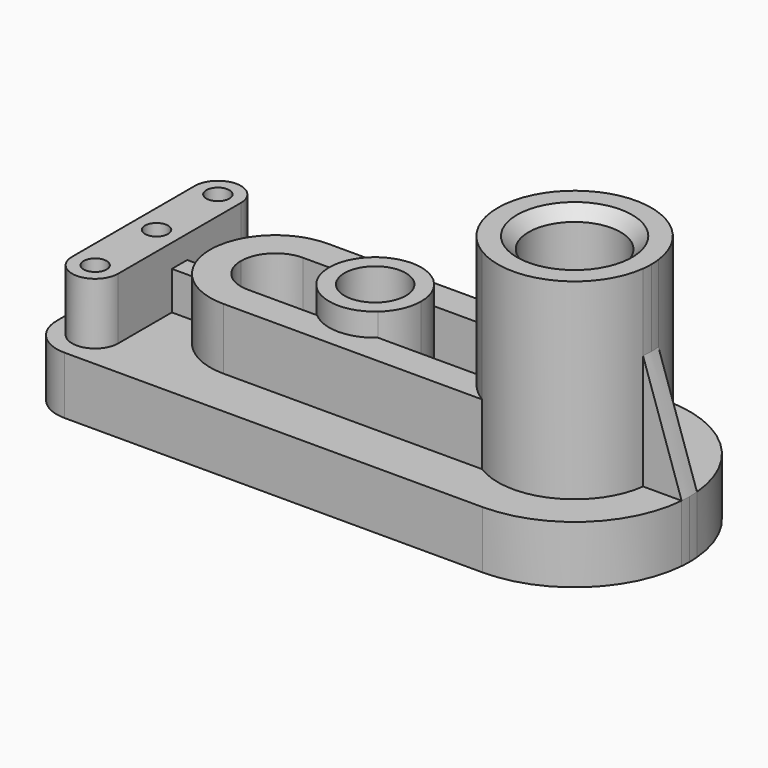
from build123d import *

# Parameters (mm, degrees)
F1_DEPTH     = 15
F0_R         = 3
F2_DEPTH     = 31
F3_DEPTH     = 25
F4_DEPTH     = 31
F5_DEPTH     = 37
F6_DEPTH     = 27
F7_DEPTH     = 65
F8_DEPTH     = 10
F9_SIZE2     = 3
F9_SIZE      = 3
F10_DEPTH    = 45
F11_T2_ANGLE = 306.9338182571


# Not quite as in the source:
# - a fillet or chamfer that OpenCascade refuses, or shapes differently, is made with other operations: its cross-section is extruded or revolved along the edge and cut away or added


with BuildPart() as f1:
    # F0 (on Top) → F1 (new body)
    with BuildSketch(Plane.XY):
        with BuildLine():
            Line((-85.9011153158, 20), (-85.9011153158, 0))
            Line((-85.9011153158, 0), (-85.9011153158, -20))
            ThreePointArc((-85.9011153158, -20), (-82.9721818815, -27.0710655334), (-75.9011153158, -29.9999964754))
            Line((-75.9011153158, -29.9999964754), (33.0988846842, -29.9999964754))
            ThreePointArc((33.0988846842, -29.9999964754), (53.399789309, -22.0744789725), (62.9799943814, -2.5))
            Line((62.9799943814, -2.5), (52.9274773566, -2.5))
            ThreePointArc((52.9274773566, -2.5), (41.6994339923, -18.0493822328), (22.5486887708, -17))
            Line((22.5486887708, -17), (-44.9011153158, -17))
            ThreePointArc((-44.9011153158, -17), (-56.0029169714, -12.8743931896), (-61.7162870366, -2.5))
            Line((-61.7162870366, -2.5), (-69.9011153158, -2.5))
            Line((-69.9011153158, -2.5), (-69.9011153158, -19.9999964754))
            ThreePointArc((-69.9011153158, -19.9999964754), (-75.9011153158, -25.9999964754), (-81.9011153158, -19.9999964754))
            Line((-81.9011153158, -19.9999964754), (-81.9011153158, 0))
            Line((-81.9011153158, 0), (-81.9011153158, 19.9999964754))
            ThreePointArc((-81.9011153158, 19.9999964754), (-75.9011153158, 25.9999964754), (-69.9011153158, 19.9999964754))
            Line((-69.9011153158, 19.9999964754), (-69.9011153158, 2.5))
            Line((-69.9011153158, 2.5), (-61.7162870366, 2.5))
            ThreePointArc((-61.7162870366, 2.5), (-56.0029169714, 12.8743931896), (-44.9011153158, 17))
            Line((-44.9011153158, 17), (22.5486887708, 17))
            ThreePointArc((22.5486887708, 17), (41.6994339923, 18.0493822328), (52.9274773566, 2.5))
            Line((52.9274773566, 2.5), (62.9799943814, 2.5))
            ThreePointArc((62.9799943814, 2.5), (53.399789309, 22.0744789725), (33.0988846842, 29.9999964754))
            Line((33.0988846842, 29.9999964754), (-75.9011153158, 29.9999964754))
            ThreePointArc((-75.9011153158, 29.9999964754), (-82.9721818815, 27.0710655334), (-85.9011153158, 20))
        make_face()
    extrude(amount=F1_DEPTH)

    # F0 (on Top) → F2 (join)
    with BuildSketch(Plane.XY):
        with BuildLine():
            Line((-69.9011153158, -19.9999964754), (-69.9011153158, -2.5))
            Line((-69.9011153158, -2.5), (-69.9011153158, 0))
            Line((-69.9011153158, 0), (-69.9011153158, 2.5))
            Line((-69.9011153158, 2.5), (-69.9011153158, 19.9999964754))
            ThreePointArc((-69.9011153158, 19.9999964754), (-75.9011153158, 25.9999964754), (-81.9011153158, 19.9999964754))
            Line((-81.9011153158, 19.9999964754), (-81.9011153158, 0))
            Line((-81.9011153158, 0), (-81.9011153158, -19.9999964754))
            ThreePointArc((-81.9011153158, -19.9999964754), (-75.9011153158, -25.9999964754), (-69.9011153158, -19.9999964754))
        make_face()
        with Locations((-75.9011153158, -19.9999964754)):
            Circle(F0_R, mode=Mode.SUBTRACT)
        with BuildLine():
            ThreePointArc((-72.9011153158, 0), (-75.9011153158, -3), (-78.9011153158, 0))
            ThreePointArc((-78.9011153158, 0), (-75.9011153158, 3), (-72.9011153158, 0))
        make_face(mode=Mode.SUBTRACT)
        with Locations((-75.9011153158, 19.9999964754)):
            Circle(F0_R, mode=Mode.SUBTRACT)
    extrude(amount=F2_DEPTH)

    # F0 (on Top) → F3 (join)
    with BuildSketch(Plane.XY):
        with BuildLine():
            Line((-69.9011153158, -2.5), (-61.7162870366, -2.5))
            ThreePointArc((-61.7162870366, -2.5), (-61.8548452778, -1.253411494), (-61.9011153158, 0))
            ThreePointArc((-61.9011153158, 0), (-61.8548452778, 1.253411494), (-61.7162870366, 2.5))
            Line((-61.7162870366, 2.5), (-69.9011153158, 2.5))
            Line((-69.9011153158, 2.5), (-69.9011153158, 0))
            Line((-69.9011153158, 0), (-69.9011153158, -2.5))
        make_face()
    extrude(amount=F3_DEPTH)


with BuildPart() as f1b:
    # F0 (on Top) → F1, piece 2 (new body)
    with BuildSketch(Plane.XY):
        with BuildLine():
            Line((-44.9011153158, -9), (-26.838369249, -9))
            ThreePointArc((-26.838369249, -9), (-29.838369249, -4.9372539332), (-30.9011153158, 0))
            ThreePointArc((-30.9011153158, 0), (-29.838369249, 4.9372539332), (-26.838369249, 9))
            Line((-26.838369249, 9), (-44.9011153158, 9))
            ThreePointArc((-44.9011153158, 9), (-51.2650763465, 6.3639610307), (-53.9011153158, 0))
            ThreePointArc((-53.9011153158, 0), (-51.2650763465, -6.3639610307), (-44.9011153158, -9))
        make_face()
    extrude(amount=F1_DEPTH)


with BuildPart() as f1c:
    # F0 (on Top) → F1, piece 3 (new body)
    with BuildSketch(Plane.XY):
        with BuildLine():
            Line((-10.9638613826, -9), (15.2237714241, -9))
            ThreePointArc((15.2237714241, -9), (13.6265494577, -4.6253960917), (13.0843425236, 0))
            ThreePointArc((13.0843425236, 0), (13.6265494577, 4.6253960917), (15.2237714241, 9))
            Line((15.2237714241, 9), (-10.9638613826, 9))
            ThreePointArc((-10.9638613826, 9), (-7.9638613826, 4.9372539332), (-6.9011153158, 0))
            ThreePointArc((-6.9011153158, 0), (-7.9638613826, -4.9372539332), (-10.9638613826, -9))
        make_face()
    extrude(amount=F1_DEPTH)


with BuildPart() as f4:
    # F0 (on Top) → F4 (new body)
    with BuildSketch(Plane.XY):
        with BuildLine():
            Line((-44.9011153158, -17), (22.5486887708, -17))
            ThreePointArc((22.5486887708, -17), (18.3335324962, -13.5060580309), (15.2237714241, -9))
            Line((15.2237714241, -9), (-10.9638613826, -9))
            ThreePointArc((-10.9638613826, -9), (-18.9011153158, -12), (-26.838369249, -9))
            Line((-26.838369249, -9), (-44.9011153158, -9))
            ThreePointArc((-44.9011153158, -9), (-51.2650763465, -6.3639610307), (-53.9011153158, 0))
            ThreePointArc((-53.9011153158, 0), (-51.2650763465, 6.3639610307), (-44.9011153158, 9))
            Line((-44.9011153158, 9), (-26.838369249, 9))
            ThreePointArc((-26.838369249, 9), (-18.9011153158, 12), (-10.9638613826, 9))
            Line((-10.9638613826, 9), (15.2237714241, 9))
            ThreePointArc((15.2237714241, 9), (18.3335324962, 13.5060580309), (22.5486887708, 17))
            Line((22.5486887708, 17), (-44.9011153158, 17))
            ThreePointArc((-44.9011153158, 17), (-56.0029169714, 12.8743931896), (-61.7162870366, 2.5))
            ThreePointArc((-61.7162870366, 2.5), (-61.8548452778, 1.253411494), (-61.9011153158, 0))
            ThreePointArc((-61.9011153158, 0), (-61.8548452778, -1.253411494), (-61.7162870366, -2.5))
            ThreePointArc((-61.7162870366, -2.5), (-56.0029169714, -12.8743931896), (-44.9011153158, -17))
        make_face()
    extrude(amount=F4_DEPTH)


with BuildPart() as f5:
    # F0 (on Top) → F5 (new body)
    with BuildSketch(Plane.XY):
        with BuildLine():
            ThreePointArc((-26.838369249, -9), (-18.9011153158, -12), (-10.9638613826, -9))
            ThreePointArc((-10.9638613826, -9), (-7.9638613826, -4.9372539332), (-6.9011153158, 0))
            ThreePointArc((-6.9011153158, 0), (-7.9638613826, 4.9372539332), (-10.9638613826, 9))
            ThreePointArc((-10.9638613826, 9), (-18.9011153158, 12), (-26.838369249, 9))
            ThreePointArc((-26.838369249, 9), (-29.838369249, 4.9372539332), (-30.9011153158, 0))
            ThreePointArc((-30.9011153158, 0), (-29.838369249, -4.9372539332), (-26.838369249, -9))
        make_face()
        with BuildLine():
            ThreePointArc((-10.9011153158, 0), (-18.9011153158, -8), (-26.9011153158, 0))
            ThreePointArc((-26.9011153158, 0), (-18.9011153158, 8), (-10.9011153158, 0))
        make_face(mode=Mode.SUBTRACT)
    extrude(amount=F5_DEPTH)

    # F0 (on Top) → F6 (join)
    with BuildSketch(Plane.XY):
        with BuildLine():
            ThreePointArc((-10.9011153158, 0), (-18.9011153158, 8), (-26.9011153158, 0))
            ThreePointArc((-26.9011153158, 0), (-18.9011153158, -8), (-10.9011153158, 0))
        make_face()
        with BuildLine():
            ThreePointArc((-13.9011153158, 0), (-18.9011153158, -5), (-23.9011153158, 0))
            ThreePointArc((-23.9011153158, 0), (-18.9011153158, 5), (-13.9011153158, 0))
        make_face(mode=Mode.SUBTRACT)
    extrude(amount=F6_DEPTH)


with BuildPart() as f7:
    # F0 (on Top) → F7 (new body)
    with BuildSketch(Plane.XY):
        with BuildLine():
            ThreePointArc((22.5486887708, -17), (41.6994339923, -18.0493822328), (52.9274773566, -2.5))
            ThreePointArc((52.9274773566, -2.5), (53.0450877084, -1.2524582509), (53.0843425236, 0))
            ThreePointArc((53.0843425236, 0), (53.0450877084, 1.2524582509), (52.9274773566, 2.5))
            ThreePointArc((52.9274773566, 2.5), (41.6994339923, 18.0493822328), (22.5486887708, 17))
            ThreePointArc((22.5486887708, 17), (18.3335324962, 13.5060580309), (15.2237714241, 9))
            ThreePointArc((15.2237714241, 9), (13.6265494577, 4.6253960917), (13.0843425236, 0))
            ThreePointArc((13.0843425236, 0), (13.6265494577, -4.6253960917), (15.2237714241, -9))
            ThreePointArc((15.2237714241, -9), (18.3335324962, -13.5060580309), (22.5486887708, -17))
        make_face()
        with BuildLine():
            ThreePointArc((49.0843425236, 0), (33.0843425236, -16), (17.0843425236, 0))
            ThreePointArc((17.0843425236, 0), (33.0843425236, 16), (49.0843425236, 0))
        make_face(mode=Mode.SUBTRACT)
        with BuildLine():
            ThreePointArc((49.0843425236, 0), (33.0843425236, 16), (17.0843425236, 0))
            ThreePointArc((17.0843425236, 0), (33.0843425236, -16), (49.0843425236, 0))
        make_face()
        with BuildLine():
            ThreePointArc((45.0843425236, 0), (33.0843425236, -12), (21.0843425236, 0))
            ThreePointArc((21.0843425236, 0), (33.0843425236, 12), (45.0843425236, 0))
        make_face(mode=Mode.SUBTRACT)
    extrude(amount=F7_DEPTH)

    # F0 (on Top) → F8 (cut)
    with BuildSketch(Plane.XY):
        with BuildLine():
            ThreePointArc((49.0843425236, 0), (33.0843425236, 16), (17.0843425236, 0))
            ThreePointArc((17.0843425236, 0), (33.0843425236, -16), (49.0843425236, 0))
        make_face()
        with BuildLine():
            ThreePointArc((45.0843425236, 0), (33.0843425236, -12), (21.0843425236, 0))
            ThreePointArc((21.0843425236, 0), (33.0843425236, 12), (45.0843425236, 0))
        make_face(mode=Mode.SUBTRACT)
    extrude(amount=F8_DEPTH, mode=Mode.SUBTRACT)

    # F9
    f9_edges = [f7.edges().sort_by_distance(p)[0] for p in [
        (45.084343, 0, 65),
    ]]
    chamfer(f9_edges, length=F9_SIZE, length2=F9_SIZE2)


with BuildPart() as f10:
    # F0 (on Top) → F10 (new body)
    with BuildSketch(Plane.XY):
        with BuildLine():
            Line((52.9274773566, -2.5), (62.9799943814, -2.5))
            ThreePointArc((62.9799943814, -2.5), (63.058244136, -1.2510883797), (63.0843425236, 0))
            ThreePointArc((63.0843425236, 0), (63.058244136, 1.2510883797), (62.9799943814, 2.5))
            Line((62.9799943814, 2.5), (52.9274773566, 2.5))
            ThreePointArc((52.9274773566, 2.5), (53.0450877084, 1.2524582509), (53.0843425236, 0))
            ThreePointArc((53.0843425236, 0), (53.0450877084, -1.2524582509), (52.9274773566, -2.5))
        make_face()
    extrude(amount=F10_DEPTH)

    # F11: chamfer of 10 x 30 on 1 edges, made by hand

    # F11_s1 → F11_t2 (revolve, cut)
    with BuildSketch(Plane(origin=(6.6021107949, 13.2226558591, 0), x_dir=(0, 0, 1), z_dir=(-0.4467146032, -0.8946765132, 0))):
        Polygon((45, -9.5997842104), (15, 0.4002157896), (45, 0.4002157896), align=None)
    revolve(axis=Axis((33.0843425236, 0, 45), (0, 0, -1)), revolution_arc=F11_T2_ANGLE, mode=Mode.SUBTRACT)


solid = Compound([f1.part, f1b.part, f1c.part, f4.part, f5.part, f7.part, f10.part])
